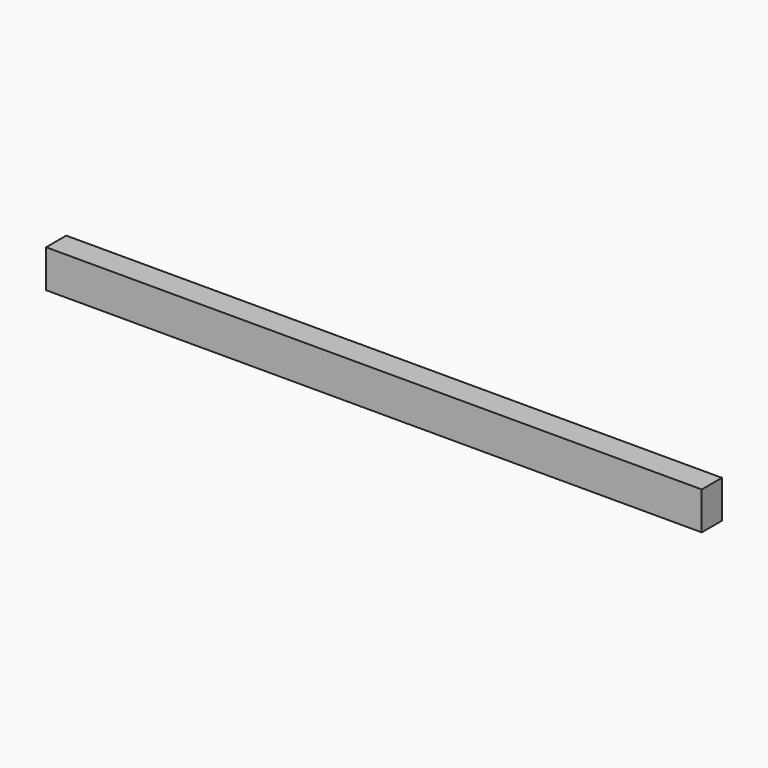
from build123d import *

# Parameters (mm, degrees)
F0_W     = 330.2
F0_H     = 19.05
F1_DEPTH = 12.7


# Not quite as in the source:
# - a feature names something its author has since deleted; it is built from what else it names


with BuildPart() as f1:
    # F0 (on Front) → F1 (new body)
    with BuildSketch(Plane.XZ):
        Rectangle(F0_W, F0_H)
    extrude(amount=F1_DEPTH)


solid = f1.part
